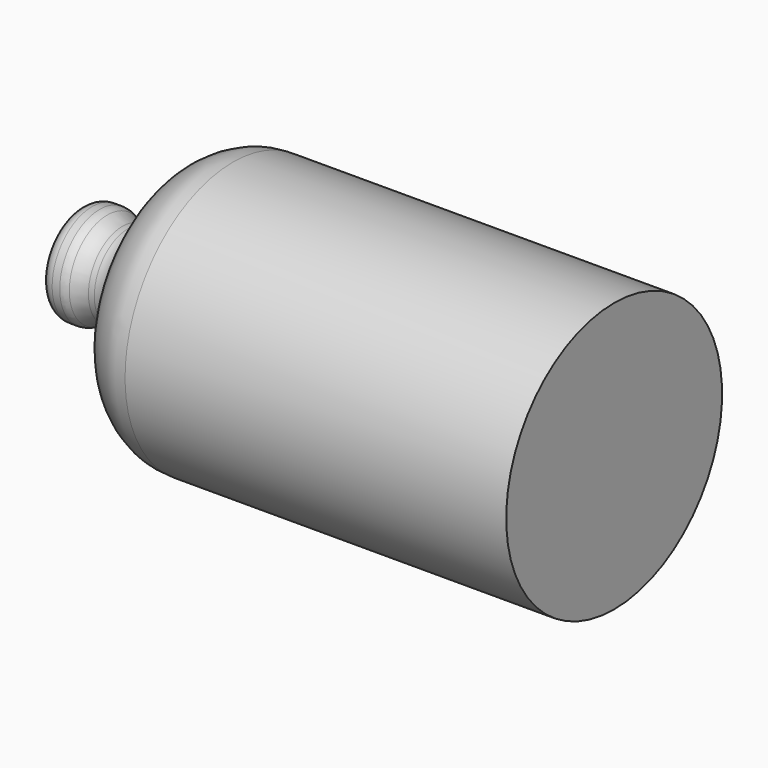
from build123d import *

# Parameters (mm, degrees)
F2_R = 12.7
F4_R = 2.54


# Not quite as in the source:
# - a fillet or chamfer that OpenCascade refuses, or shapes differently, is made with other operations: its cross-section is extruded or revolved along the edge and cut away or added


with BuildPart() as f1:
    # F0 (on Front) → F1 (revolve)
    with BuildSketch(Plane.XZ):
        Polygon((53.5, 27), (-30.1052267423, 27), (-40.7862067223, 8.5), (-48.5, 8.5), (-48.5, 10), (-53.5, 10), (-53.5, 6.5), (-39.6315061839, 6.5), (-28.9505262039, 25), (51.5, 25), (51.5, 0), (53.5, 0), align=None)
    revolve(axis=Axis((0, 0, 0), (1, 0, 0)))

    # F2
    f2_edges = [f1.edges().sort_by_distance(p)[0] for p in [
        (-30.105227, 0, -27),
        (-28.950526, 0, -25),
    ]]
    fillet(f2_edges, radius=F2_R)

    # F3: fillet of radius 5.08 on 2 edges, made by hand

    # F3_s1 → F3_t2 (revolve)
    with BuildSketch(Plane.XZ):
        with BuildLine():
            ThreePointArc((-43.7191460897, 8.5), (-41.1791460897, 9.1805909488), (-39.3197370385, 11.04))
            Line((-39.3197370385, 11.04), (-40.7862067223, 8.5))
            Line((-40.7862067223, 8.5), (-43.7191460897, 8.5))
        make_face()
    revolve(axis=Axis((-40.7862067223, 0, 0), (1, 0, 0)))

    # F3_s3 → F3_t4 (revolve)
    with BuildSketch(Plane.XZ):
        with BuildLine():
            ThreePointArc((-48.5, 10), (-46.8477578714, 8.8899680172), (-44.8958357418, 8.5))
            Line((-44.8958357418, 8.5), (-48.5, 8.5))
            Line((-48.5, 8.5), (-48.5, 10))
        make_face()
    revolve(axis=Axis((-48.5, 0, 0), (1, 0, 0)))

    # F4
    f4_edges = [f1.edges().sort_by_distance(p)[0] for p in [
        (-48.5, 0, -10),
        (-53.5, 0, -10),
    ]]
    fillet(f4_edges, radius=F4_R)

    # F5: fillet of radius 2.54 on 1 edges, made by hand

    # F5_s1 → F5_t2 (revolve, cut)
    with BuildSketch(Plane.XZ):
        with BuildLine():
            ThreePointArc((-53.5, 7.46), (-52.6154054362, 6.7525560116), (-51.5112315369, 6.5))
            Line((-51.5112315369, 6.5), (-53.5, 6.5))
            Line((-53.5, 6.5), (-53.5, 7.46))
        make_face()
    revolve(axis=Axis((-53.5, 0, 0), (1, 0, 0)), mode=Mode.SUBTRACT)


solid = f1.part
